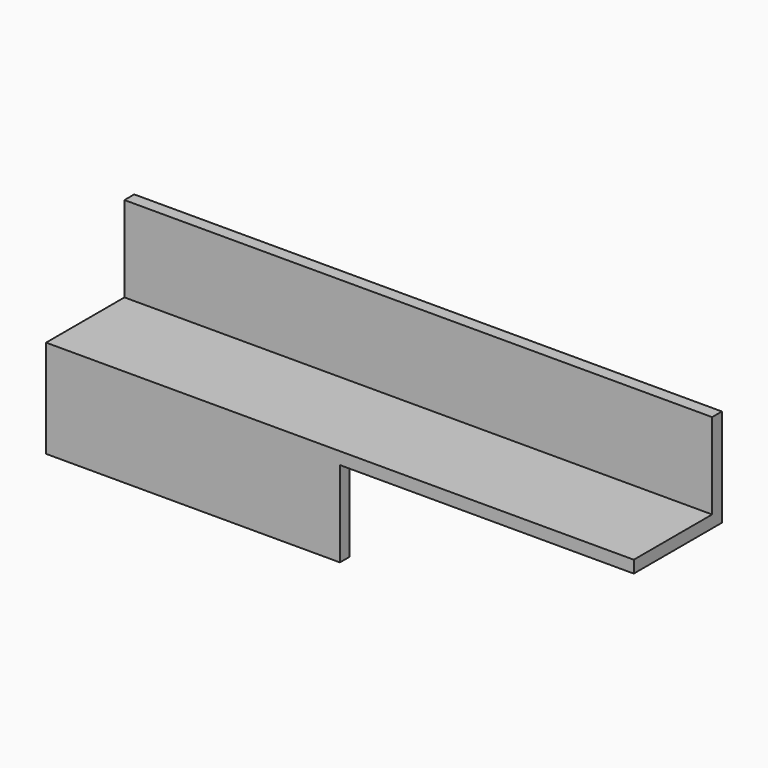
from build123d import *

# Parameters (mm, degrees)
F0_W     = 152.4
F0_H     = 25.4
F1_DEPTH = 3.175
F2_W     = 25.4
F2_H     = 3.175
F3_DEPTH = 152.4
F4_W     = 76.2
F4_H     = 22.225
F5_DEPTH = 3.175


# Not quite as in the source:
# - a length typed as a fraction of an inch, garbled in the dataset ("3 / 203.2 mm" for 3/8 in), is restored


with BuildPart() as f1:
    # F0 (on Front) → F1 (new body)
    with BuildSketch(Plane.XZ):
        with Locations((48.1263138257, 41.5133684874)):
            Rectangle(F0_W, F0_H)
    extrude(amount=F1_DEPTH)

    # F2 (on face) → F3 (join)
    with BuildSketch(Plane.YZ.offset(124.3263138257)):
        with Locations((-15.875, 30.4008684874)):
            Rectangle(F2_W, F2_H)
    extrude(amount=-F3_DEPTH)

    # F4 (on face) → F5 (join)
    with BuildSketch(Plane.XZ.offset(28.575)):
        with Locations((10.0263138257, 17.7008684874)):
            Rectangle(F4_W, F4_H)
    extrude(amount=-F5_DEPTH)


solid = f1.part
